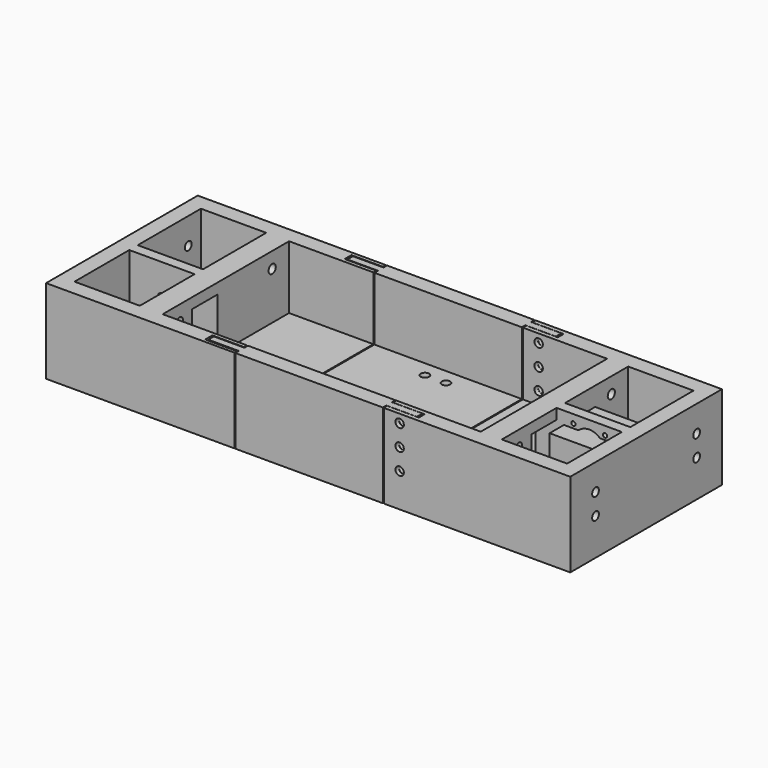
from build123d import *

# Parameters (mm, degrees)
F0_W           = 48
F0_H           = 54
F1_DEPTH       = 48
F2_R           = 5.4958473914
F3_DEPTH       = 28
F4_W           = 62
F4_H           = 10
F5_DEPTH       = 60
F6_W           = 62
F6_H           = 75
F6_H_2         = 65
F6_W_2         = 80
F6_H_3         = 150
F7_DEPTH       = 20
F8_W           = 30
F8_H           = 40
F9_DEPTH       = 25
F10_R          = 2
F10_R_2        = 15
F11_DEPTH      = 25
F11_DEPTH_BACK = 25
F13_R          = 4
F15_DEPTH      = 25
F17_DEPTH      = 60
F14_W          = 30
F14_H          = 7
F18_DEPTH      = 62
F12_R          = 4
F19_DEPTH      = 300
F21_W          = 70
F21_H          = 165
F22_DEPTH      = 20
F24_W          = 62
F24_H          = 10
F25_DEPTH      = 60
F26_W          = 62
F26_H          = 75
F26_H_2        = 65
F26_W_2        = 80
F26_H_3        = 150
F26_W_3        = 30
F26_H_4        = 8.5
F26_H_5        = 8
F27_DEPTH      = 20
F28_R          = 4
F29_DEPTH      = 25
F30_W          = 30
F30_H          = 40
F31_DEPTH      = 25
F32_R          = 4
F33_DEPTH      = 25
F34_R          = 4.25
F35_DEPTH      = 25
F36_R          = 4.25
F37_DEPTH      = 25
F38_R          = 4
F39_DEPTH      = 25


# Not quite as in the source:
# - a feature names something its author has since deleted; it is built from what else it names


with BuildPart() as f1:
    # F0 (on Top) → F1 (new body)
    with BuildSketch(Plane.XY):
        Rectangle(F0_W, F0_H)
    extrude(amount=F1_DEPTH)

    # F2 (on face) → F3 (join)
    with BuildSketch(Plane.XZ.offset(27)):
        with Locations((0, 24)):
            Circle(F2_R)
    extrude(amount=F3_DEPTH)


with BuildPart() as f5:
    # F4 (on Top) → F5 (new body)
    with BuildSketch(Plane.XY):
        Polygon((31, -10), (31, -75), (-31, -75), (-51, -75), (-131, -75), (-131, -90), (46, -90), (46, 90), (-131, 90), (-131, 75), (-51, 75), (-31, 75), (31, 75), (31, 0), align=None)
        Polygon((-51, -75), (-31, -75), (-31, -10), (-31, 0), (-31, 75), (-51, 75), (-51, 74.3744149804), align=None)
        with Locations((0, -5)):
            Rectangle(F4_W, F4_H)
    extrude(amount=F5_DEPTH)

    # F6 (on face) → F7 (join)
    with BuildSketch(Plane(origin=(0, 0, 0), x_dir=(1, 0, 0), z_dir=(0, 0, -1))):
        Polygon((46, -90), (46, 90), (-131, 90), (-131, 75), (-51, 75), (-51, -75), (-131, -75), (-131, -90), align=None)
        with Locations((0, -37.5)):
            Rectangle(F6_W, F6_H, mode=Mode.SUBTRACT)
        with Locations((0, 42.5)):
            Rectangle(F6_W, F6_H_2, mode=Mode.SUBTRACT)
        with Locations((-91, 0)):
            Rectangle(F6_W_2, F6_H_3)
        with Locations((0, -37.5)):
            Rectangle(F6_W, F6_H)
        with Locations((0, 42.5)):
            Rectangle(F6_W, F6_H_2)
    extrude(amount=F7_DEPTH)

    # F8 (on face) → F9 (cut)
    with BuildSketch(Plane.YZ.offset(-31)):
        with Locations((-25, 30)):
            Rectangle(F8_W, F8_H)
    extrude(amount=-F9_DEPTH, mode=Mode.SUBTRACT)

    # F10 (on face) → F11 (cut, two sides)
    with BuildSketch(Plane.XZ.offset(10)) as f11_sk:
        with Locations((-15, 52)):
            Circle(F10_R)
        with Locations((15, 52)):
            Circle(F10_R)
        with Locations((-15, 22)):
            Circle(F10_R)
        with Locations((15, 22)):
            Circle(F10_R)
        with Locations((0, 37)):
            Circle(F10_R_2)
    extrude(amount=-F11_DEPTH, mode=Mode.SUBTRACT)
    extrude(f11_sk.sketch, amount=F11_DEPTH_BACK, mode=Mode.SUBTRACT)

    # F13 (on face) → F15 (cut)
    with BuildSketch(Plane.YZ.offset(46)):
        with Locations((-60, 15)):
            Circle(F13_R)
        with Locations((-60, 35)):
            Circle(F13_R)
        with Locations((60, 35)):
            Circle(F13_R)
        with Locations((60, 15)):
            Circle(F13_R)
    extrude(amount=-F15_DEPTH, mode=Mode.SUBTRACT)

    # F14 (on face) → F18 (cut)
    with BuildSketch(Plane.XY.offset(60)):
        with Locations((-116, -82.5)):
            Rectangle(F14_W, F14_H)
        with Locations((-116, 82.5)):
            Rectangle(F14_W, F14_H)
    extrude(amount=-F18_DEPTH, mode=Mode.SUBTRACT)


with BuildPart() as f17:
    # F16 (on Top) → F17 (new body)
    with BuildSketch(Plane.XY):
        Polygon((-202, -90), (-132, -90), (-132, -85.8), (-103, -85.8), (-103, -79.2), (-132, -79.2), (-132, -75), (-202, -75), align=None)
    extrude(amount=F17_DEPTH)


with BuildPart() as f19_tool:
    # F12 (on face) → F19 (new body)
    with BuildSketch(Plane.XZ.offset(90)):
        with Locations((-116, 12)):
            Circle(F12_R)
        with Locations((-116, 32)):
            Circle(F12_R)
        with Locations((-116, 52)):
            Circle(F12_R)
    extrude(amount=-F19_DEPTH)


with BuildPart() as f5_1:
    add(f5.part)

    # F19: cut by f19_tool
    add(f19_tool.part, mode=Mode.SUBTRACT)

    # F36 (on face) → F37 (cut)
    with BuildSketch(Plane(origin=(-51, 0, 0), x_dir=(0, -1, 0), z_dir=(-1, 0, 0))):
        with Locations((55, 45)):
            Circle(F36_R)
        with Locations((-55, 45)):
            Circle(F36_R)
    extrude(amount=-F37_DEPTH, mode=Mode.SUBTRACT)


with BuildPart() as f17_1:
    add(f17.part)

    # F19: cut by f19_tool
    add(f19_tool.part, mode=Mode.SUBTRACT)


with BuildPart() as f20_1:
    # F20: instance of F17
    add(f17_1.part.mirror(Plane.XZ))


with BuildPart() as f17_2:
    add(f17_1.part)

    add(f20_1.part)  # F22 merges F20_1
    # F21 (on face) → F22 (join)
    with BuildSketch(Plane(origin=(0, 0, 0), x_dir=(1, 0, 0), z_dir=(0, 0, -1))):
        Polygon((-132, 90), (-202, 90), (-202, 75), (-132, 75), (-132, 79.2), (-132, 85.8), align=None)
        with Locations((-167, -7.5)):
            Rectangle(F21_W, F21_H)
    extrude(amount=F22_DEPTH)

    # F23: F17 across face


with BuildPart() as f17_3:
    add(f17_2.part)
    add(f17_2.part.mirror(Plane(origin=(-202, 0, 3.3333333333), x_dir=(0, -1, 0), z_dir=(-1, 0, 0))))

    # F38 (on face) → F39 (cut)
    with BuildSketch(Plane.XY):
        with Locations((-212, 60)):
            Circle(F38_R)
        with Locations((-192, -60)):
            Circle(F38_R)
        with Locations((-212, -60)):
            Circle(F38_R)
        with Locations((-192, 60)):
            Circle(F38_R)
    extrude(amount=-F39_DEPTH, mode=Mode.SUBTRACT)


with BuildPart() as f25:
    # F24 (on Top) → F25 (new body)
    with BuildSketch(Plane.XY):
        Polygon((-353, -90), (-273, -90), (-273, -87), (-303, -87), (-303, -78.5), (-273, -78.5), (-273, -75), (-353, -75), (-374.6794085503, -75), (-436.6794085503, -75), (-436.6794085503, -10), (-436.6794085503, 0), (-436.6794085503, 75), (-374.6794085503, 75), (-353, 75), (-273, 75), (-273, 78.5), (-303, 78.5), (-303, 86.5), (-273, 86.5), (-273, 90), (-353, 90), (-374.6794085503, 90), (-436.6794085503, 90), (-451.6794085503, 90), (-451.6794085503, -90), (-436.6794085503, -90), (-374.6794085503, -90), align=None)
        Polygon((-374.6794085503, -75), (-353, -75), (-353, 75), (-374.6794085503, 75), (-374.6794085503, 0), (-374.6794085503, -10), align=None)
        with Locations((-405.6794085503, -5)):
            Rectangle(F24_W, F24_H)
    extrude(amount=F25_DEPTH)

    # F26 (on face) → F27 (join)
    with BuildSketch(Plane(origin=(0, 0, 0), x_dir=(1, 0, 0), z_dir=(0, 0, -1))):
        Polygon((-451.6794085503, 87), (-451.6794085503, -90), (-273, -90), (-273, -86.5), (-303, -86.5), (-303, -78.5), (-273, -78.5), (-273, -75), (-353, -75), (-353, 75), (-273, 75), (-273, 78.5), (-303, 78.5), (-303, 87), align=None)
        with Locations((-405.6794085503, -37.5)):
            Rectangle(F26_W, F26_H, mode=Mode.SUBTRACT)
        with Locations((-405.6794085503, 42.5)):
            Rectangle(F26_W, F26_H_2, mode=Mode.SUBTRACT)
        Polygon((-451.6794085503, 90), (-451.6794085503, 87), (-303, 87), (-273, 87), (-273, 90), align=None)
        with Locations((-405.6794085503, -37.5)):
            Rectangle(F26_W, F26_H)
        with Locations((-405.6794085503, 42.5)):
            Rectangle(F26_W, F26_H_2)
        with Locations((-313, 0)):
            Rectangle(F26_W_2, F26_H_3)
        with Locations((-288, 82.75)):
            Rectangle(F26_W_3, F26_H_4)
        with Locations((-288, -82.5)):
            Rectangle(F26_W_3, F26_H_5)
    extrude(amount=F27_DEPTH)

    # F28 (on face) → F29 (cut)
    with BuildSketch(Plane.XZ.offset(10)):
        with Locations((-405.6794085503, 30)):
            Circle(F28_R)
    extrude(amount=-F29_DEPTH, mode=Mode.SUBTRACT)

    # F30 (on face) → F31 (cut)
    with BuildSketch(Plane(origin=(-374.6794085503, 0, 0), x_dir=(0, -1, 0), z_dir=(-1, 0, 0))):
        with Locations((25, 30)):
            Rectangle(F30_W, F30_H)
    extrude(amount=-F31_DEPTH, mode=Mode.SUBTRACT)

    # F32 (on face) → F33 (cut)
    with BuildSketch(Plane(origin=(-451.6794085503, 0, 0), x_dir=(0, -1, 0), z_dir=(-1, 0, 0))):
        with Locations((60, 35)):
            Circle(F32_R)
        with Locations((60, 15)):
            Circle(F32_R)
        with Locations((-60, 35)):
            Circle(F32_R)
        with Locations((-60, 15)):
            Circle(F32_R)
    extrude(amount=-F33_DEPTH, mode=Mode.SUBTRACT)

    # F34 (on face) → F35 (cut)
    with BuildSketch(Plane.YZ.offset(-353)):
        with Locations((55, 45)):
            Circle(F34_R)
        with Locations((-55, 45)):
            Circle(F34_R)
    extrude(amount=-F35_DEPTH, mode=Mode.SUBTRACT)


solid = Compound([f1.part, f5_1.part, f17_3.part, f25.part])
